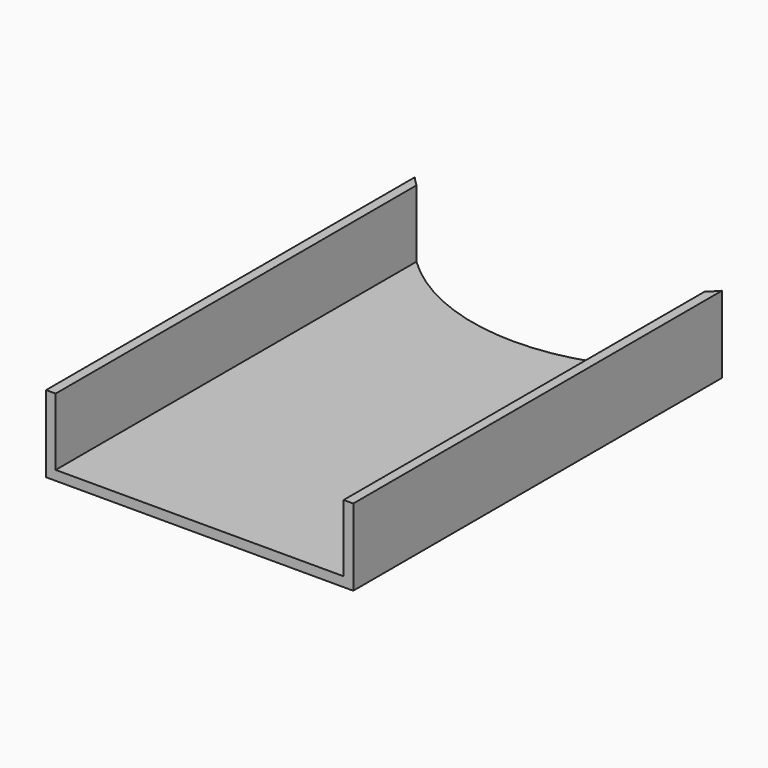
from build123d import *

# Parameters (mm, degrees)
F1_DEPTH = 3.175
F2_DEPTH = 25.4
F3_DEPTH = 25.4


with BuildPart() as f1:
    # F0 (on Top) → F1 (new body)
    with BuildSketch(Plane.XY):
        with BuildLine():
            ThreePointArc((98.425, 149.3462514694), (50.8, 130.1850769842), (3.175, 149.3462514694))
            Line((3.175, 149.3462514694), (3.175, 3.3780224621))
            Line((3.175, 3.3780224621), (3.175, 0.2030224621))
            Line((3.175, 0.2030224621), (98.425, 0.2030224621))
            Line((98.425, 0.2030224621), (98.425, 3.3780224621))
            Line((98.425, 3.3780224621), (98.425, 149.3462514694))
        make_face()
    extrude(amount=F1_DEPTH)

    # F0 (on Top) → F2 (join)
    with BuildSketch(Plane.XY):
        with BuildLine():
            ThreePointArc((3.175, 149.3462514694), (1.5605666607, 150.9483798686), (0, 152.6030224621))
            Line((0, 152.6030224621), (0, 0.2030224621))
            Line((0, 0.2030224621), (3.175, 0.2030224621))
            Line((3.175, 0.2030224621), (3.175, 3.3780224621))
            Line((3.175, 3.3780224621), (3.175, 149.3462514694))
        make_face()
    extrude(amount=F2_DEPTH)

    # F0 (on Top) → F3 (join)
    with BuildSketch(Plane.XY):
        with BuildLine():
            ThreePointArc((101.6, 152.6030224621), (100.0394333393, 150.9483798686), (98.425, 149.3462514694))
            Line((98.425, 149.3462514694), (98.425, 3.3780224621))
            Line((98.425, 3.3780224621), (98.425, 0.2030224621))
            Line((98.425, 0.2030224621), (101.6, 0.2030224621))
            Line((101.6, 0.2030224621), (101.6, 152.6030224621))
        make_face()
    extrude(amount=F3_DEPTH)


solid = f1.part
